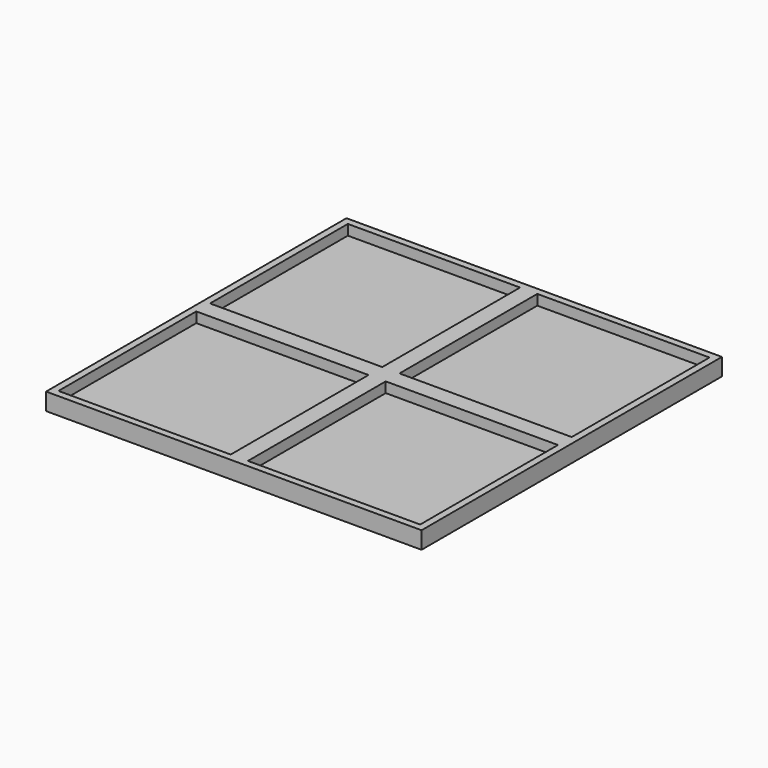
from build123d import *

# Parameters (mm, degrees)
F0_W     = 109
F0_H     = 109
F0_W_2   = 5
F0_H_2   = 5
F0_W_3   = 50
F0_H_3   = 50
F1_DEPTH = 2
F2_DEPTH = 5


with BuildPart() as f1:
    # F0 (on Top) → F1 (new body)
    with BuildSketch(Plane.XY):
        Rectangle(F0_W, F0_H)
        Polygon((-2.5, -52.5), (-52.5, -52.5), (-52.5, -2.5), (-52.5, 2.5), (-52.5, 52.5), (-2.5, 52.5), (2.5, 52.5), (52.5, 52.5), (52.5, 2.5), (52.5, -2.5), (52.5, -52.5), (2.5, -52.5), align=None, mode=Mode.SUBTRACT)
        Rectangle(F0_W_2, F0_H_2)
        with Locations((-27.5, 27.5)):
            Rectangle(F0_W_3, F0_H_3)
        with Locations((-27.5, -27.5)):
            Rectangle(F0_W_3, F0_H_3)
        with Locations((27.5, -27.5)):
            Rectangle(F0_W_3, F0_H_3)
        with Locations((27.5, 27.5)):
            Rectangle(F0_W_3, F0_H_3)
        with Locations((0, 27.5)):
            Rectangle(F0_W_2, F0_H_3)
        with Locations((27.5, 0)):
            Rectangle(F0_W_3, F0_H_2)
        with Locations((0, -27.5)):
            Rectangle(F0_W_2, F0_H_3)
        with Locations((-27.5, 0)):
            Rectangle(F0_W_3, F0_H_2)
    extrude(amount=F1_DEPTH)

    # F0 (on Top) → F2 (join)
    with BuildSketch(Plane.XY):
        Rectangle(F0_W, F0_H)
        Polygon((-2.5, -52.5), (-52.5, -52.5), (-52.5, -2.5), (-52.5, 2.5), (-52.5, 52.5), (-2.5, 52.5), (2.5, 52.5), (52.5, 52.5), (52.5, 2.5), (52.5, -2.5), (52.5, -52.5), (2.5, -52.5), align=None, mode=Mode.SUBTRACT)
        with Locations((0, -27.5)):
            Rectangle(F0_W_2, F0_H_3)
        with Locations((27.5, 0)):
            Rectangle(F0_W_3, F0_H_2)
        with Locations((-27.5, 0)):
            Rectangle(F0_W_3, F0_H_2)
        with Locations((0, 27.5)):
            Rectangle(F0_W_2, F0_H_3)
        Rectangle(F0_W_2, F0_H_2)
    extrude(amount=F2_DEPTH)


solid = f1.part
